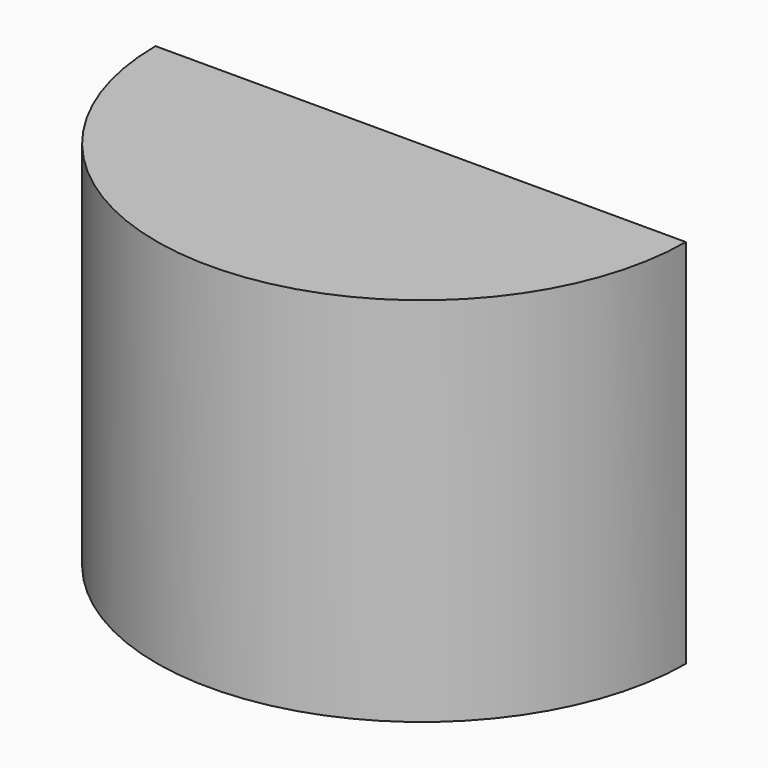
from build123d import *

# Parameters (mm, degrees)
F1_DEPTH = 15.875
F2_DEPTH = 0.79375
F4_DEPTH = 0.79375
F6_DEPTH = 5.08


# Not quite as in the source:
# - a length typed as a fraction of an inch, garbled in the dataset ("3 / 203.2 mm" for 3/8 in), is restored


with BuildPart() as f1:
    # F0 (on Top) → F1 (new body)
    with BuildSketch(Plane.XY):
        with BuildLine():
            Line((-5.732164003, 16.9486273388), (-8.1134518534, 16.9486273388))
            ThreePointArc((-8.1134518534, 16.9486273388), (3.7927981466, 5.1022697967), (15.6990481466, 16.9486273388))
            Line((15.6990481466, 16.9486273388), (13.3177602962, 16.9486273388))
            ThreePointArc((13.3177602962, 16.9486273388), (3.7927981466, 7.4835197967), (-5.732164003, 16.9486273388))
        make_face()
    extrude(amount=F1_DEPTH)

    # F0 (on Top) → F2 (join)
    with BuildSketch(Plane.XY):
        with BuildLine():
            Line((13.3177602962, 16.9486273388), (-5.732164003, 16.9486273388))
            ThreePointArc((-5.732164003, 16.9486273388), (3.7927981466, 7.4835197967), (13.3177602962, 16.9486273388))
        make_face()
    extrude(amount=F2_DEPTH)

    # F3 (on face) → F4 (join)
    with BuildSketch(Plane.XY.offset(15.875)):
        with BuildLine():
            Line((13.3177602962, 16.9486273388), (-5.732164003, 16.9486273388))
            ThreePointArc((-5.732164003, 16.9486273388), (3.7927981466, 7.4236651892), (13.3177602962, 16.9486273388))
        make_face()
        with BuildLine():
            ThreePointArc((13.3177602962, 16.9486273388), (3.7927981466, 7.4236651892), (-5.732164003, 16.9486273388))
            Line((-5.732164003, 16.9486273388), (-8.1134518534, 16.9486273388))
            ThreePointArc((-8.1134518534, 16.9486273388), (3.7927981466, 5.1022697967), (15.6990481466, 16.9486273388))
            Line((15.6990481466, 16.9486273388), (13.3177602962, 16.9486273388))
        make_face()
    extrude(amount=F4_DEPTH)

    # F5 (on face) → F6 (cut)
    with BuildSketch(Plane(origin=(0, 0, 0), x_dir=(1, 0, 0), z_dir=(0, 0, -1))):
        with BuildLine():
            ThreePointArc((6.1740481466, -16.9486273388), (3.7927981466, -14.5673773388), (1.4115481466, -16.9486273388))
            Line((1.4115481466, -16.9486273388), (6.1740481466, -16.9486273388))
        make_face()
    extrude(amount=-F6_DEPTH, mode=Mode.SUBTRACT)


solid = f1.part
